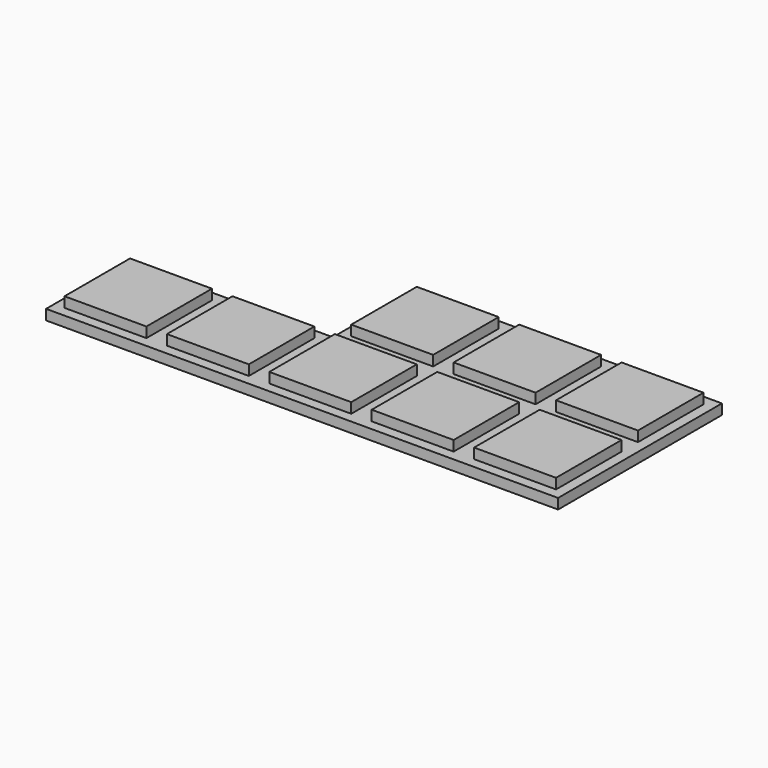
from build123d import *

# Parameters (mm, degrees)
F1_DEPTH = 1
F2_W     = 8
F2_H     = 8
F3_DEPTH = 1


# Not quite as in the source:
# - a feature names something its author has since deleted; it is built from what else it names


with BuildPart() as f1:
    # F0 (on Top) → F1 (new body)
    with BuildSketch(Plane.XY):
        Polygon((-3.6520181931, 1.5305465425), (-23.6520181931, 1.5305465425), (-23.6520181931, -8.4694534575), (26.3479818069, -8.4694534575), (26.3479818069, 11.5305465425), (-3.6520181931, 11.5305465425), align=None)
    extrude(amount=F1_DEPTH)

    # F2 (on face) → F3 (join)
    with BuildSketch(Plane.XY.offset(1)):
        with Locations((-18.6520181931, -3.4694534575)):
            Rectangle(F2_W, F2_H)
        with Locations((-8.6520181931, -3.4694534575)):
            Rectangle(F2_W, F2_H)
        with Locations((1.3479818069, 6.5305465425)):
            Rectangle(F2_W, F2_H)
        with Locations((11.3479818069, 6.5305465425)):
            Rectangle(F2_W, F2_H)
        with Locations((11.3479818069, -3.4694534575)):
            Rectangle(F2_W, F2_H)
        with Locations((21.3479818069, -3.4694534575)):
            Rectangle(F2_W, F2_H)
        with Locations((21.3479818069, 6.5305465425)):
            Rectangle(F2_W, F2_H)
        with Locations((1.3479818069, -3.4694534575)):
            Rectangle(F2_W, F2_H)
    extrude(amount=F3_DEPTH)


solid = f1.part
